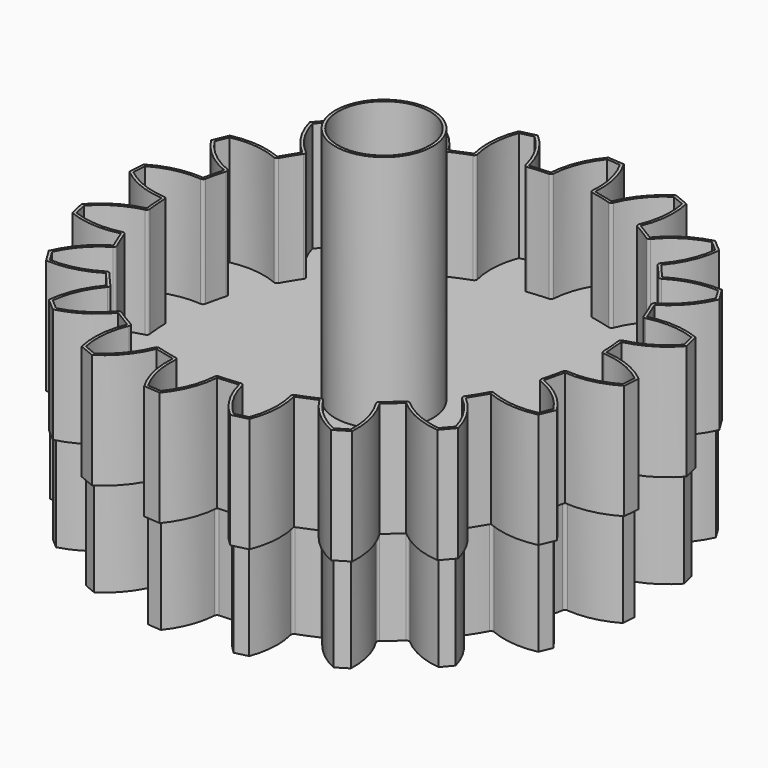
from build123d import *

# Parameters (mm, degrees)
F3_DEPTH  = 10
F5_COUNT  = 20
F5_ANGLE  = 342
F6_R      = 22.4
F6_R_2    = 4.8
F7_DEPTH  = 10
F9_DEPTH  = 12
F10_DEPTH = 0.5
F11_R     = 5.1
F11_R_2   = 4.8
F12_DEPTH = 25


with BuildPart() as f3:
    # F2 (on Top) → F3 (new body)
    with BuildSketch(Plane.XY):
        with BuildLine():
            ThreePointArc((-0.3948414618, 22.6683412707), (-0.4862144866, 22.4730928102), (-0.6849292807, 22.3895259414))
            ThreePointArc((-0.6849292807, 22.3895259414), (1.7574837443, 22.3309482756), (4.1789901778, 22.0067271782))
            ThreePointArc((4.1789901778, 22.0067271782), (3.995794631, 22.1203510427), (3.9360901482, 22.3274895609))
            ThreePointArc((3.9360901482, 22.3274895609), (3.7716615062, 24.8715195619), (2.8560164403, 27.25074623))
            Line((2.8560164403, 27.25074623), (1.4421017698, 27.3620237279))
            ThreePointArc((1.4421017698, 27.3620237279), (0.165536763, 25.1553277343), (-0.3948414618, 22.6683412707))
        make_face()
    extrude(amount=F3_DEPTH)


with BuildPart() as f5_1:
    # F5: instance of F3
    add(f3.part.rotate(Axis((0, 0, 7.5), (0, 0, 1)), 1 * F5_ANGLE / (F5_COUNT - 1)))


with BuildPart() as f5_2:
    # F5: instance of F3
    add(f3.part.rotate(Axis((0, 0, 7.5), (0, 0, 1)), 2 * F5_ANGLE / (F5_COUNT - 1)))


with BuildPart() as f5_3:
    # F5: instance of F3
    add(f3.part.rotate(Axis((0, 0, 7.5), (0, 0, 1)), 3 * F5_ANGLE / (F5_COUNT - 1)))


with BuildPart() as f5_4:
    # F5: instance of F3
    add(f3.part.rotate(Axis((0, 0, 7.5), (0, 0, 1)), 4 * F5_ANGLE / (F5_COUNT - 1)))


with BuildPart() as f5_5:
    # F5: instance of F3
    add(f3.part.rotate(Axis((0, 0, 7.5), (0, 0, 1)), 5 * F5_ANGLE / (F5_COUNT - 1)))


with BuildPart() as f5_6:
    # F5: instance of F3
    add(f3.part.rotate(Axis((0, 0, 7.5), (0, 0, 1)), 6 * F5_ANGLE / (F5_COUNT - 1)))


with BuildPart() as f5_7:
    # F5: instance of F3
    add(f3.part.rotate(Axis((0, 0, 7.5), (0, 0, 1)), 7 * F5_ANGLE / (F5_COUNT - 1)))


with BuildPart() as f5_8:
    # F5: instance of F3
    add(f3.part.rotate(Axis((0, 0, 7.5), (0, 0, 1)), 8 * F5_ANGLE / (F5_COUNT - 1)))


with BuildPart() as f5_9:
    # F5: instance of F3
    add(f3.part.rotate(Axis((0, 0, 7.5), (0, 0, 1)), 9 * F5_ANGLE / (F5_COUNT - 1)))


with BuildPart() as f5_10:
    # F5: instance of F3
    add(f3.part.rotate(Axis((0, 0, 7.5), (0, 0, 1)), 10 * F5_ANGLE / (F5_COUNT - 1)))


with BuildPart() as f5_11:
    # F5: instance of F3
    add(f3.part.rotate(Axis((0, 0, 7.5), (0, 0, 1)), 11 * F5_ANGLE / (F5_COUNT - 1)))


with BuildPart() as f5_12:
    # F5: instance of F3
    add(f3.part.rotate(Axis((0, 0, 7.5), (0, 0, 1)), 12 * F5_ANGLE / (F5_COUNT - 1)))


with BuildPart() as f5_13:
    # F5: instance of F3
    add(f3.part.rotate(Axis((0, 0, 7.5), (0, 0, 1)), 13 * F5_ANGLE / (F5_COUNT - 1)))


with BuildPart() as f5_14:
    # F5: instance of F3
    add(f3.part.rotate(Axis((0, 0, 7.5), (0, 0, 1)), 14 * F5_ANGLE / (F5_COUNT - 1)))


with BuildPart() as f5_15:
    # F5: instance of F3
    add(f3.part.rotate(Axis((0, 0, 7.5), (0, 0, 1)), 15 * F5_ANGLE / (F5_COUNT - 1)))


with BuildPart() as f5_16:
    # F5: instance of F3
    add(f3.part.rotate(Axis((0, 0, 7.5), (0, 0, 1)), 16 * F5_ANGLE / (F5_COUNT - 1)))


with BuildPart() as f5_17:
    # F5: instance of F3
    add(f3.part.rotate(Axis((0, 0, 7.5), (0, 0, 1)), 17 * F5_ANGLE / (F5_COUNT - 1)))


with BuildPart() as f5_18:
    # F5: instance of F3
    add(f3.part.rotate(Axis((0, 0, 7.5), (0, 0, 1)), 18 * F5_ANGLE / (F5_COUNT - 1)))


with BuildPart() as f5_19:
    # F5: instance of F3
    add(f3.part.rotate(Axis((0, 0, 7.5), (0, 0, 1)), 19 * F5_ANGLE / (F5_COUNT - 1)))


with BuildPart() as f3_1:
    add(f3.part)

    add(f5_1.part)  # F7 merges F5_1

    add(f5_2.part)  # F7 merges F5_2

    add(f5_3.part)  # F7 merges F5_3

    add(f5_4.part)  # F7 merges F5_4

    add(f5_5.part)  # F7 merges F5_5

    add(f5_6.part)  # F7 merges F5_6

    add(f5_7.part)  # F7 merges F5_7

    add(f5_8.part)  # F7 merges F5_8

    add(f5_9.part)  # F7 merges F5_9

    add(f5_10.part)  # F7 merges F5_10

    add(f5_11.part)  # F7 merges F5_11

    add(f5_12.part)  # F7 merges F5_12

    add(f5_13.part)  # F7 merges F5_13

    add(f5_14.part)  # F7 merges F5_14

    add(f5_15.part)  # F7 merges F5_15

    add(f5_16.part)  # F7 merges F5_16

    add(f5_17.part)  # F7 merges F5_17

    add(f5_18.part)  # F7 merges F5_18

    add(f5_19.part)  # F7 merges F5_19
    # F6 (on Top) → F7 (join)
    with BuildSketch(Plane.XY):
        Circle(F6_R)
        Circle(F6_R_2, mode=Mode.SUBTRACT)
    extrude(amount=F7_DEPTH)


with BuildPart() as f9:
    # F8 (on face) → F9 (new body)
    with BuildSketch(Plane.XY.offset(10)):
        with BuildLine():
            Line((3.0360651894, 27.5375037457), (1.3091284782, 27.6734166124))
            ThreePointArc((1.3091284782, 27.6734166124), (-0.0843791365, 25.3389143017), (-0.6941024407, 22.6893856638))
            Line((-0.6941024407, 22.6893856638), (-2.8638450205, 22.5186232194))
            ThreePointArc((-2.8638450205, 22.5186232194), (-3.8805392142, 25.0401500242), (-5.6220870578, 27.1279181194))
            Line((-5.6220870578, 27.1279181194), (-7.3065008558, 26.723526145))
            ThreePointArc((-7.3065008558, 26.723526145), (-7.9104044658, 24.0726649754), (-7.6715364113, 21.3643986363))
            Line((-7.6715364113, 21.3643986363), (-9.6823157332, 20.5315065702))
            ThreePointArc((-9.6823157332, 20.5315065702), (-11.4284440056, 22.615445285), (-13.7299102524, 24.0628628562))
            Line((-13.7299102524, 24.0628628562), (-15.2069189787, 23.1577507447))
            ThreePointArc((-15.2069189787, 23.1577507447), (-14.962104291, 20.4500154771), (-13.8980269471, 17.9481154157))
            Line((-13.8980269471, 17.9481154157), (-15.5530139212, 16.5346230065))
            ThreePointArc((-15.5530139212, 16.5346230065), (-17.8576530711, 17.9769831902), (-20.4937541696, 18.6423669209))
            Line((-20.4937541696, 18.6423669209), (-21.6187779191, 17.325133352))
            ThreePointArc((-21.6187779191, 17.325133352), (-20.5492091011, 14.8255759803), (-18.7640817722, 12.7749456064))
            Line((-18.7640817722, 12.7749456064), (-19.9012747424, 10.9192153394))
            ThreePointArc((-19.9012747424, 10.9192153394), (-22.5388306324, 11.5788087278), (-25.2515266403, 11.3970262223))
            Line((-25.2515266403, 11.3970262223), (-25.9144402498, 9.7966111955))
            ThreePointArc((-25.9144402498, 9.7966111955), (-24.1248141496, 7.7499058107), (-21.7933775363, 6.3512751128))
            Line((-21.7933775363, 6.3512751128), (-22.3014601314, 4.2349587963))
            ThreePointArc((-22.3014601314, 4.2349587963), (-25.0137504141, 4.0472197928), (-27.5375037457, 3.0360651894))
            Line((-27.5375037457, 3.0360651894), (-27.6734166124, 1.3091284782))
            ThreePointArc((-27.6734166124, 1.3091284782), (-25.3389143017, -0.0843791365), (-22.6893856638, -0.6941024407))
            Line((-22.6893856638, -0.6941024407), (-22.5186232194, -2.8638450205))
            ThreePointArc((-22.5186232194, -2.8638450205), (-25.0401500242, -3.8805392142), (-27.1279181194, -5.6220870578))
            Line((-27.1279181194, -5.6220870578), (-26.723526145, -7.3065008558))
            ThreePointArc((-26.723526145, -7.3065008558), (-24.0726649754, -7.9104044658), (-21.3643986363, -7.6715364113))
            Line((-21.3643986363, -7.6715364113), (-20.5315065702, -9.6823157332))
            ThreePointArc((-20.5315065702, -9.6823157332), (-22.615445285, -11.4284440056), (-24.0628628562, -13.7299102524))
            Line((-24.0628628562, -13.7299102524), (-23.1577507447, -15.2069189787))
            ThreePointArc((-23.1577507447, -15.2069189787), (-20.4500154771, -14.962104291), (-17.9481154157, -13.8980269471))
            Line((-17.9481154157, -13.8980269471), (-16.5346230065, -15.5530139212))
            ThreePointArc((-16.5346230065, -15.5530139212), (-17.9769831902, -17.8576530711), (-18.6423669209, -20.4937541696))
            Line((-18.6423669209, -20.4937541696), (-17.325133352, -21.6187779191))
            ThreePointArc((-17.325133352, -21.6187779191), (-14.8255759803, -20.5492091011), (-12.7749456064, -18.7640817722))
            Line((-12.7749456064, -18.7640817722), (-10.9192153394, -19.9012747424))
            ThreePointArc((-10.9192153394, -19.9012747424), (-11.5788087278, -22.5388306324), (-11.3970262223, -25.2515266403))
            Line((-11.3970262223, -25.2515266403), (-9.7966111955, -25.9144402498))
            ThreePointArc((-9.7966111955, -25.9144402498), (-7.7499058107, -24.1248141496), (-6.3512751128, -21.7933775363))
            Line((-6.3512751128, -21.7933775363), (-4.2349587963, -22.3014601314))
            ThreePointArc((-4.2349587963, -22.3014601314), (-4.0472197928, -25.0137504141), (-3.0360651894, -27.5375037457))
            Line((-3.0360651894, -27.5375037457), (-1.3091284782, -27.6734166124))
            ThreePointArc((-1.3091284782, -27.6734166124), (0.0843791365, -25.3389143017), (0.6941024407, -22.6893856638))
            Line((0.6941024407, -22.6893856638), (2.8638450205, -22.5186232194))
            ThreePointArc((2.8638450205, -22.5186232194), (3.8805392142, -25.0401500242), (5.6220870578, -27.1279181194))
            Line((5.6220870578, -27.1279181194), (7.3065008558, -26.723526145))
            ThreePointArc((7.3065008558, -26.723526145), (7.9104044658, -24.0726649754), (7.6715364113, -21.3643986363))
            Line((7.6715364113, -21.3643986363), (9.6823157332, -20.5315065702))
            ThreePointArc((9.6823157332, -20.5315065702), (11.4284440056, -22.615445285), (13.7299102524, -24.0628628562))
            Line((13.7299102524, -24.0628628562), (15.2069189787, -23.1577507447))
            ThreePointArc((15.2069189787, -23.1577507447), (14.962104291, -20.4500154771), (13.8980269471, -17.9481154157))
            Line((13.8980269471, -17.9481154157), (15.5530139212, -16.5346230065))
            ThreePointArc((15.5530139212, -16.5346230065), (17.8576530711, -17.9769831902), (20.4937541696, -18.6423669209))
            Line((20.4937541696, -18.6423669209), (21.6187779191, -17.325133352))
            ThreePointArc((21.6187779191, -17.325133352), (20.5492091011, -14.8255759803), (18.7640817722, -12.7749456064))
            Line((18.7640817722, -12.7749456064), (19.9012747424, -10.9192153394))
            ThreePointArc((19.9012747424, -10.9192153394), (22.5388306324, -11.5788087278), (25.2515266403, -11.3970262223))
            Line((25.2515266403, -11.3970262223), (25.9144402498, -9.7966111955))
            ThreePointArc((25.9144402498, -9.7966111955), (24.1248141496, -7.7499058107), (21.7933775363, -6.3512751128))
            Line((21.7933775363, -6.3512751128), (22.3014601314, -4.2349587963))
            ThreePointArc((22.3014601314, -4.2349587963), (25.0137504141, -4.0472197928), (27.5375037457, -3.0360651894))
            Line((27.5375037457, -3.0360651894), (27.6734166124, -1.3091284782))
            ThreePointArc((27.6734166124, -1.3091284782), (25.3389143017, 0.0843791365), (22.6893856638, 0.6941024407))
            Line((22.6893856638, 0.6941024407), (22.5186232194, 2.8638450205))
            ThreePointArc((22.5186232194, 2.8638450205), (25.0401500242, 3.8805392142), (27.1279181194, 5.6220870578))
            Line((27.1279181194, 5.6220870578), (26.723526145, 7.3065008558))
            ThreePointArc((26.723526145, 7.3065008558), (24.0726649754, 7.9104044658), (21.3643986363, 7.6715364113))
            Line((21.3643986363, 7.6715364113), (20.5315065702, 9.6823157332))
            ThreePointArc((20.5315065702, 9.6823157332), (22.615445285, 11.4284440056), (24.0628628562, 13.7299102524))
            Line((24.0628628562, 13.7299102524), (23.1577507447, 15.2069189787))
            ThreePointArc((23.1577507447, 15.2069189787), (20.4500154771, 14.962104291), (17.9481154157, 13.8980269471))
            Line((17.9481154157, 13.8980269471), (16.5346230065, 15.5530139212))
            ThreePointArc((16.5346230065, 15.5530139212), (17.9769831902, 17.8576530711), (18.6423669209, 20.4937541696))
            Line((18.6423669209, 20.4937541696), (17.325133352, 21.6187779191))
            ThreePointArc((17.325133352, 21.6187779191), (14.8255759803, 20.5492091011), (12.7749456064, 18.7640817722))
            Line((12.7749456064, 18.7640817722), (10.9192153394, 19.9012747424))
            ThreePointArc((10.9192153394, 19.9012747424), (11.5788087278, 22.5388306324), (11.3970262223, 25.2515266403))
            Line((11.3970262223, 25.2515266403), (9.7966111955, 25.9144402498))
            ThreePointArc((9.7966111955, 25.9144402498), (7.7499058107, 24.1248141496), (6.3512751128, 21.7933775363))
            Line((6.3512751128, 21.7933775363), (4.2349587963, 22.3014601314))
            ThreePointArc((4.2349587963, 22.3014601314), (4.0472197928, 25.0137504141), (3.0360651894, 27.5375037457))
        make_face()
        with BuildLine():
            ThreePointArc((-0.3948414618, 22.6683412707), (0.165536763, 25.1553277343), (1.4421017698, 27.3620237279))
            Line((1.4421017698, 27.3620237279), (2.8560164403, 27.25074623))
            ThreePointArc((2.8560164403, 27.25074623), (3.7716615062, 24.8715195619), (3.9360901482, 22.3274895609))
            ThreePointArc((3.9360901482, 22.3274895609), (3.995794631, 22.1203510427), (4.1789901778, 22.0067271782))
            ThreePointArc((4.1789901778, 22.0067271782), (5.2291761504, 21.7810862169), (6.2673375563, 21.505359331))
            ThreePointArc((6.2673375563, 21.505359331), (6.4821501388, 21.5234298977), (6.6293861418, 21.6808864009))
            ThreePointArc((6.6293861418, 21.6808864009), (7.9308585861, 23.8729846882), (9.8268506177, 25.577197011))
            Line((9.8268506177, 25.577197011), (11.1371767407, 25.0344421597))
            ThreePointArc((11.1371767407, 25.0344421597), (11.2727854733, 22.4887132471), (10.6430179002, 20.0183856922))
            ThreePointArc((10.6430179002, 20.0183856922), (10.6357909153, 19.8029355549), (10.7749085288, 19.6382623008))
            ThreePointArc((10.7749085288, 19.6382623008), (11.7039678496, 19.0991396815), (12.6061137261, 18.5160983126))
            ThreePointArc((12.6061137261, 18.5160983126), (12.8159967447, 18.4669037043), (13.0046832402, 18.5711553105))
            ThreePointArc((13.0046832402, 18.5711553105), (14.9198527133, 20.2537875681), (17.2496788595, 21.2886960438))
            Line((17.2496788595, 21.2886960438), (18.3281525844, 20.3675924655))
            ThreePointArc((18.3281525844, 20.3675924655), (17.6704506562, 17.9045549915), (16.3081329059, 15.7497427557))
            ThreePointArc((16.3081329059, 15.7497427557), (16.2346818809, 15.5470707598), (16.3161037597, 15.3474674817))
            ThreePointArc((16.3161037597, 15.3474674817), (17.0330936294, 14.5476362826), (17.7109156525, 13.7143525822))
            ThreePointArc((17.7109156525, 13.7143525822), (17.895324295, 13.6027083098), (18.1069913341, 13.6435501455))
            ThreePointArc((18.1069913341, 13.6435501455), (20.4483877041, 14.6520086043), (22.9839883489, 14.9163091808))
            Line((22.9839883489, 14.9163091808), (23.7250411534, 13.7070209115))
            ThreePointArc((23.7250411534, 13.7070209115), (22.3384090115, 11.567774145), (20.3768942373, 9.9394052633))
            ThreePointArc((20.3768942373, 9.9394052633), (20.2444090703, 9.7693503559), (20.2601650737, 9.5543556134))
            ThreePointArc((20.2601650737, 9.5543556134), (20.6949015283, 8.572108885), (21.0820497556, 7.5701504675))
            ThreePointArc((21.0820497556, 7.5701504675), (21.2229328192, 7.4069850503), (21.4368609573, 7.380419232))
            ThreePointArc((21.4368609573, 7.380419232), (23.9752920342, 7.6159889518), (26.4684649199, 7.0838100471))
            Line((26.4684649199, 7.0838100471), (26.7995573922, 5.7047106482))
            ThreePointArc((26.7995573922, 5.7047106482), (24.819728252, 4.0986589678), (22.4510231865, 3.1561295319))
            ThreePointArc((22.4510231865, 3.1561295319), (22.2724724489, 3.0353378722), (22.2210202694, 2.8259968485))
            ThreePointArc((22.2210202694, 2.8259968485), (22.3309482756, 1.7574837443), (22.3895259414, 0.6849292807))
            ThreePointArc((22.3895259414, 0.6849292807), (22.4730928102, 0.4862144866), (22.6683412707, 0.3948414618))
            ThreePointArc((22.6683412707, 0.3948414618), (25.1553277343, -0.165536763), (27.3620237279, -1.4421017698))
            Line((27.3620237279, -1.4421017698), (27.25074623, -2.8560164403))
            ThreePointArc((27.25074623, -2.8560164403), (24.8715195619, -3.7716615062), (22.3274895609, -3.9360901482))
            ThreePointArc((22.3274895609, -3.9360901482), (22.1203510427, -3.995794631), (22.0067271782, -4.1789901778))
            ThreePointArc((22.0067271782, -4.1789901778), (21.7810862169, -5.2291761504), (21.505359331, -6.2673375563))
            ThreePointArc((21.505359331, -6.2673375563), (21.5234298977, -6.4821501388), (21.6808864009, -6.6293861418))
            ThreePointArc((21.6808864009, -6.6293861418), (23.8729846882, -7.9308585861), (25.577197011, -9.8268506177))
            Line((25.577197011, -9.8268506177), (25.0344421597, -11.1371767407))
            ThreePointArc((25.0344421597, -11.1371767407), (22.4887132471, -11.2727854733), (20.0183856922, -10.6430179002))
            ThreePointArc((20.0183856922, -10.6430179002), (19.8029355549, -10.6357909153), (19.6382623008, -10.7749085288))
            ThreePointArc((19.6382623008, -10.7749085288), (19.0991396815, -11.7039678496), (18.5160983126, -12.6061137261))
            ThreePointArc((18.5160983126, -12.6061137261), (18.4669037043, -12.8159967447), (18.5711553105, -13.0046832402))
            ThreePointArc((18.5711553105, -13.0046832402), (20.2537875681, -14.9198527133), (21.2886960438, -17.2496788595))
            Line((21.2886960438, -17.2496788595), (20.3675924655, -18.3281525844))
            ThreePointArc((20.3675924655, -18.3281525844), (17.9045549915, -17.6704506562), (15.7497427557, -16.3081329059))
            ThreePointArc((15.7497427557, -16.3081329059), (15.5470707598, -16.2346818809), (15.3474674817, -16.3161037597))
            ThreePointArc((15.3474674817, -16.3161037597), (14.5476362826, -17.0330936294), (13.7143525822, -17.7109156525))
            ThreePointArc((13.7143525822, -17.7109156525), (13.6027083098, -17.895324295), (13.6435501455, -18.1069913341))
            ThreePointArc((13.6435501455, -18.1069913341), (14.6520086043, -20.4483877041), (14.9163091808, -22.9839883489))
            Line((14.9163091808, -22.9839883489), (13.7070209115, -23.7250411534))
            ThreePointArc((13.7070209115, -23.7250411534), (11.567774145, -22.3384090115), (9.9394052633, -20.3768942373))
            ThreePointArc((9.9394052633, -20.3768942373), (9.7693503559, -20.2444090703), (9.5543556134, -20.2601650737))
            ThreePointArc((9.5543556134, -20.2601650737), (8.572108885, -20.6949015283), (7.5701504675, -21.0820497556))
            ThreePointArc((7.5701504675, -21.0820497556), (7.4069850503, -21.2229328192), (7.380419232, -21.4368609573))
            ThreePointArc((7.380419232, -21.4368609573), (7.6159889518, -23.9752920342), (7.0838100471, -26.4684649199))
            Line((7.0838100471, -26.4684649199), (5.7047106482, -26.7995573922))
            ThreePointArc((5.7047106482, -26.7995573922), (4.0986589678, -24.819728252), (3.1561295319, -22.4510231865))
            ThreePointArc((3.1561295319, -22.4510231865), (3.0353378722, -22.2724724489), (2.8259968485, -22.2210202694))
            ThreePointArc((2.8259968485, -22.2210202694), (1.7574837443, -22.3309482756), (0.6849292807, -22.3895259414))
            ThreePointArc((0.6849292807, -22.3895259414), (0.4862144866, -22.4730928102), (0.3948414618, -22.6683412707))
            ThreePointArc((0.3948414618, -22.6683412707), (-0.165536763, -25.1553277343), (-1.4421017698, -27.3620237279))
            Line((-1.4421017698, -27.3620237279), (-2.8560164403, -27.25074623))
            ThreePointArc((-2.8560164403, -27.25074623), (-3.7716615062, -24.8715195619), (-3.9360901482, -22.3274895609))
            ThreePointArc((-3.9360901482, -22.3274895609), (-3.995794631, -22.1203510427), (-4.1789901778, -22.0067271782))
            ThreePointArc((-4.1789901778, -22.0067271782), (-5.2291761504, -21.7810862169), (-6.2673375563, -21.505359331))
            ThreePointArc((-6.2673375563, -21.505359331), (-6.4821501388, -21.5234298977), (-6.6293861418, -21.6808864009))
            ThreePointArc((-6.6293861418, -21.6808864009), (-7.9308585861, -23.8729846882), (-9.8268506177, -25.577197011))
            Line((-9.8268506177, -25.577197011), (-11.1371767407, -25.0344421597))
            ThreePointArc((-11.1371767407, -25.0344421597), (-11.2727854733, -22.4887132471), (-10.6430179002, -20.0183856922))
            ThreePointArc((-10.6430179002, -20.0183856922), (-10.6357909153, -19.8029355549), (-10.7749085288, -19.6382623008))
            ThreePointArc((-10.7749085288, -19.6382623008), (-11.7039678496, -19.0991396815), (-12.6061137261, -18.5160983126))
            ThreePointArc((-12.6061137261, -18.5160983126), (-12.8159967447, -18.4669037043), (-13.0046832402, -18.5711553105))
            ThreePointArc((-13.0046832402, -18.5711553105), (-14.9198527133, -20.2537875681), (-17.2496788595, -21.2886960438))
            Line((-17.2496788595, -21.2886960438), (-18.3281525844, -20.3675924655))
            ThreePointArc((-18.3281525844, -20.3675924655), (-17.6704506562, -17.9045549915), (-16.3081329059, -15.7497427557))
            ThreePointArc((-16.3081329059, -15.7497427557), (-16.2346818809, -15.5470707598), (-16.3161037597, -15.3474674817))
            ThreePointArc((-16.3161037597, -15.3474674817), (-17.0330936294, -14.5476362826), (-17.7109156525, -13.7143525822))
            ThreePointArc((-17.7109156525, -13.7143525822), (-17.895324295, -13.6027083098), (-18.1069913341, -13.6435501455))
            ThreePointArc((-18.1069913341, -13.6435501455), (-20.4483877041, -14.6520086043), (-22.9839883489, -14.9163091808))
            Line((-22.9839883489, -14.9163091808), (-23.7250411534, -13.7070209115))
            ThreePointArc((-23.7250411534, -13.7070209115), (-22.3384090115, -11.567774145), (-20.3768942373, -9.9394052633))
            ThreePointArc((-20.3768942373, -9.9394052633), (-20.2444090703, -9.7693503559), (-20.2601650737, -9.5543556134))
            ThreePointArc((-20.2601650737, -9.5543556134), (-20.6949015283, -8.572108885), (-21.0820497556, -7.5701504675))
            ThreePointArc((-21.0820497556, -7.5701504675), (-21.2229328192, -7.4069850503), (-21.4368609573, -7.380419232))
            ThreePointArc((-21.4368609573, -7.380419232), (-23.9752920342, -7.6159889518), (-26.4684649199, -7.0838100471))
            Line((-26.4684649199, -7.0838100471), (-26.7995573922, -5.7047106482))
            ThreePointArc((-26.7995573922, -5.7047106482), (-24.819728252, -4.0986589678), (-22.4510231865, -3.1561295319))
            ThreePointArc((-22.4510231865, -3.1561295319), (-22.2724724489, -3.0353378722), (-22.2210202694, -2.8259968485))
            ThreePointArc((-22.2210202694, -2.8259968485), (-22.3309482756, -1.7574837443), (-22.3895259414, -0.6849292807))
            ThreePointArc((-22.3895259414, -0.6849292807), (-22.4730928102, -0.4862144866), (-22.6683412707, -0.3948414618))
            ThreePointArc((-22.6683412707, -0.3948414618), (-25.1553277343, 0.165536763), (-27.3620237279, 1.4421017698))
            Line((-27.3620237279, 1.4421017698), (-27.25074623, 2.8560164403))
            ThreePointArc((-27.25074623, 2.8560164403), (-24.8715195619, 3.7716615062), (-22.3274895609, 3.9360901482))
            ThreePointArc((-22.3274895609, 3.9360901482), (-22.1203510427, 3.995794631), (-22.0067271782, 4.1789901778))
            ThreePointArc((-22.0067271782, 4.1789901778), (-21.7810862169, 5.2291761504), (-21.505359331, 6.2673375563))
            ThreePointArc((-21.505359331, 6.2673375563), (-21.5234298977, 6.4821501388), (-21.6808864009, 6.6293861418))
            ThreePointArc((-21.6808864009, 6.6293861418), (-23.8729846882, 7.9308585861), (-25.577197011, 9.8268506177))
            Line((-25.577197011, 9.8268506177), (-25.0344421597, 11.1371767407))
            ThreePointArc((-25.0344421597, 11.1371767407), (-22.4887132471, 11.2727854733), (-20.0183856922, 10.6430179002))
            ThreePointArc((-20.0183856922, 10.6430179002), (-19.8029355549, 10.6357909153), (-19.6382623008, 10.7749085288))
            ThreePointArc((-19.6382623008, 10.7749085288), (-19.0991396815, 11.7039678496), (-18.5160983126, 12.6061137261))
            ThreePointArc((-18.5160983126, 12.6061137261), (-18.4669037043, 12.8159967447), (-18.5711553105, 13.0046832402))
            ThreePointArc((-18.5711553105, 13.0046832402), (-20.2537875681, 14.9198527133), (-21.2886960438, 17.2496788595))
            Line((-21.2886960438, 17.2496788595), (-20.3675924655, 18.3281525844))
            ThreePointArc((-20.3675924655, 18.3281525844), (-17.9045549915, 17.6704506562), (-15.7497427557, 16.3081329059))
            ThreePointArc((-15.7497427557, 16.3081329059), (-15.5470707598, 16.2346818809), (-15.3474674817, 16.3161037597))
            ThreePointArc((-15.3474674817, 16.3161037597), (-14.5476362826, 17.0330936294), (-13.7143525822, 17.7109156525))
            ThreePointArc((-13.7143525822, 17.7109156525), (-13.6027083098, 17.895324295), (-13.6435501455, 18.1069913341))
            ThreePointArc((-13.6435501455, 18.1069913341), (-14.6520086043, 20.4483877041), (-14.9163091808, 22.9839883489))
            Line((-14.9163091808, 22.9839883489), (-13.7070209115, 23.7250411534))
            ThreePointArc((-13.7070209115, 23.7250411534), (-11.567774145, 22.3384090115), (-9.9394052633, 20.3768942373))
            ThreePointArc((-9.9394052633, 20.3768942373), (-9.7693503559, 20.2444090703), (-9.5543556134, 20.2601650737))
            ThreePointArc((-9.5543556134, 20.2601650737), (-8.572108885, 20.6949015283), (-7.5701504675, 21.0820497556))
            ThreePointArc((-7.5701504675, 21.0820497556), (-7.4069850503, 21.2229328192), (-7.380419232, 21.4368609573))
            ThreePointArc((-7.380419232, 21.4368609573), (-7.6159889518, 23.9752920342), (-7.0838100471, 26.4684649199))
            Line((-7.0838100471, 26.4684649199), (-5.7047106482, 26.7995573922))
            ThreePointArc((-5.7047106482, 26.7995573922), (-4.0986589678, 24.819728252), (-3.1561295319, 22.4510231865))
            ThreePointArc((-3.1561295319, 22.4510231865), (-3.0353378722, 22.2724724489), (-2.8259968485, 22.2210202694))
            ThreePointArc((-2.8259968485, 22.2210202694), (-1.7574837443, 22.3309482756), (-0.6849292807, 22.3895259414))
            ThreePointArc((-0.6849292807, 22.3895259414), (-0.4862144866, 22.4730928102), (-0.3948414618, 22.6683412707))
        make_face(mode=Mode.SUBTRACT)
    extrude(amount=F9_DEPTH)

    # F10 (add): a face of the model
    f10_faces = [f3_1.part.faces().sort_by_distance(p)[0] for p in [
        (5.0485093047, 21.0285546462, 10),
    ]]
    extrude(f10_faces, amount=F10_DEPTH)

    # F11 (on face) → F12 (join)
    with BuildSketch(Plane.XY.offset(10.5)):
        Circle(F11_R)
        Circle(F11_R_2, mode=Mode.SUBTRACT)
    extrude(amount=F12_DEPTH)


solid = Compound([f3_1.part, f9.part])
